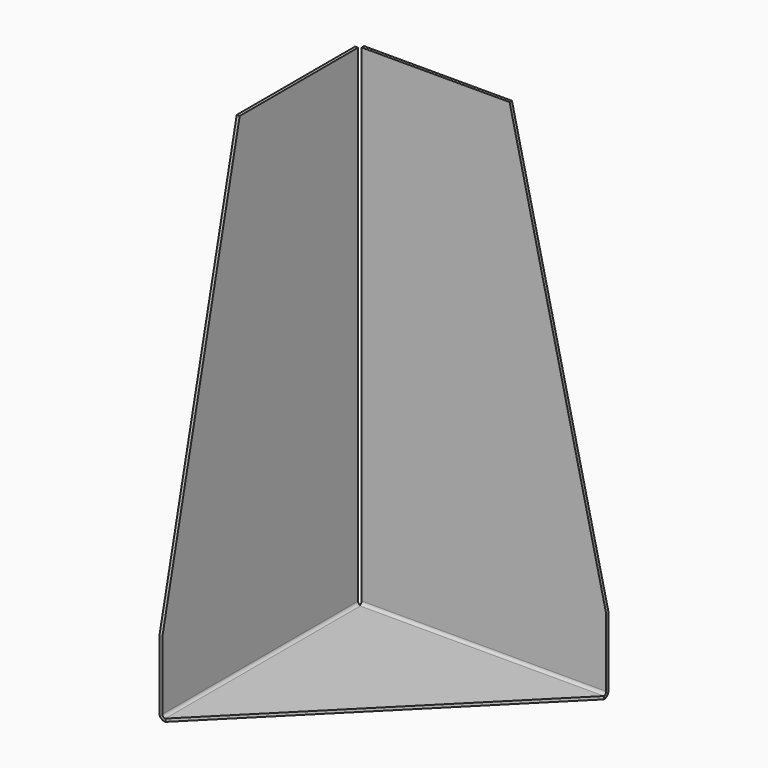
from build123d import *

# Parameters (mm, degrees)
F0_W        = 101.2
F0_H        = 101.2
F1_DEPTH    = 200
F2_T        = -1.2
F4_W        = 0.8
F4_H        = 0.8
F5_DEPTH    = 200.001
F6_R        = 1.2
F7_T4_DEPTH = 101.8
F8_R        = 2.4
F9_T1_DEPTH = 110.8
F12_DEPTH   = 25
F13_DEPTH   = 25
F15_DEPTH   = 25


# Not quite as in the source:
# - a fillet or chamfer that OpenCascade refuses, or shapes differently, is made with other operations: its cross-section is extruded or revolved along the edge and cut away or added


with BuildPart() as f1:
    # F0 (on Top) → F1 (new body)
    with BuildSketch(Plane.XY):
        Rectangle(F0_W, F0_H)
    extrude(amount=F1_DEPTH)

    # F2
    f2_openings = [f1.faces().sort_by_distance(p)[0] for p in [
        (0, 0, 200),
        (0, -50.6, 100),
        (50.6, 0, 100),
    ]]
    offset(amount=F2_T, openings=f2_openings)

    # F4 (on face) → F5 (cut, through all)
    with BuildSketch(Plane.XY.offset(200)):
        with Locations((-49, 49)):
            Rectangle(F4_W, F4_H)
        Polygon((-50.6, 50.6), (-50.6, 48.6), (-49.4, 48.6), (-49.4, 49.4), (-48.6, 49.4), (-48.6, 50.6), align=None)
    extrude(amount=-F5_DEPTH, mode=Mode.SUBTRACT)

    # F6
    f6_edges = [f1.edges().sort_by_distance(p)[0] for p in [
        (1, 49.4, 1.2),
    ]]
    fillet(f6_edges, radius=F6_R)

    # F7: fillet of radius 1.2 on 1 edges, made by hand


with BuildPart() as f7_tool2:
    # F7_s3 → F7_t4 (new body)
    with BuildSketch(Plane.XZ.offset(50.6)):
        with BuildLine():
            ThreePointArc((-49.4, 2.4), (-49.0485281374, 1.5514718626), (-48.2, 1.2))
            Line((-48.2, 1.2), (-49.4, 1.2))
            Line((-49.4, 1.2), (-49.4, 2.4))
        make_face()
    extrude(amount=-F7_T4_DEPTH)

    split(bisect_by=Plane.XZ.offset(-48.6), keep=Keep.TOP)


with BuildPart() as f1_1:
    add(f1.part)

    # F7_t1: union F7_tool2
    add(f7_tool2.part)

    # F8
    f8_edges = [f1_1.edges().sort_by_distance(p)[0] for p in [
        (-50.6, -1, 0),
    ]]
    fillet(f8_edges, radius=F8_R)

    # F9: fillet of radius 2.4 on 1 edges, made by hand

    # F9_s2 → F9_t1 (cut)
    with BuildSketch(Plane.YZ.offset(-54.2)):
        with BuildLine():
            ThreePointArc((50.6, 2.4), (49.8970562748, 0.7029437252), (48.2, 0))
            Line((48.2, 0), (50.6, 0))
            Line((50.6, 0), (50.6, 2.4))
        make_face()
    extrude(amount=F9_T1_DEPTH, mode=Mode.SUBTRACT)

    # F11 (on face) → F12 (cut)
    with BuildSketch(Plane(origin=(0, 50.6, 0), x_dir=(-1, 0, 0), z_dir=(0, 1, 0))):
        Polygon((-11.4, 200), (-50.6, 200), (-50.6, 30), align=None)
    extrude(amount=-F12_DEPTH, mode=Mode.SUBTRACT)

    # F10 (on face) → F13 (cut)
    with BuildSketch(Plane(origin=(-50.6, 0, 0), x_dir=(0, -1, 0), z_dir=(-1, 0, 0))):
        Polygon((50.6, 30), (50.6, 200), (11.4, 200), align=None)
    extrude(amount=-F13_DEPTH, mode=Mode.SUBTRACT)

    # F14 (on face) → F15 (cut)
    with BuildSketch(Plane(origin=(0, 0, 0), x_dir=(1, 0, 0), z_dir=(0, 0, -1))):
        Polygon((50.6, -48.2), (50.6, 50.6), (-48.2, 50.6), align=None)
    extrude(amount=-F15_DEPTH, mode=Mode.SUBTRACT)


solid = f1_1.part
